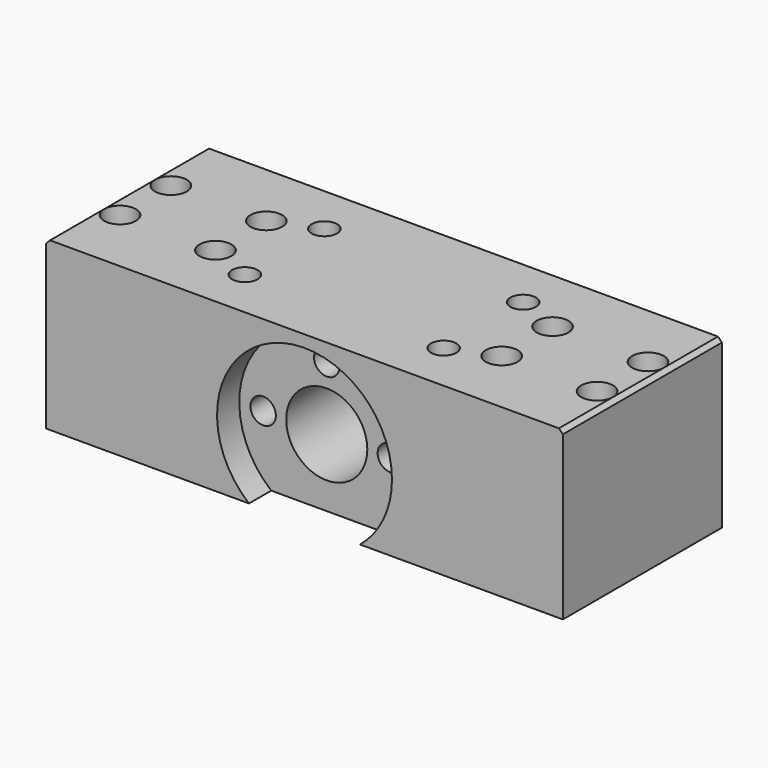
from build123d import *

# Parameters (mm, degrees)
F0_W           = 65
F0_H           = 21
F0_R           = 5.1
F1_DEPTH       = 25
F3_D           = 2.4
F3_CBORE_D     = 4
F3_CBORE_DEPTH = 2.5
F4_SIZE        = 0.49999
F5_R           = 5.1
F6_DEPTH       = 3.5
F8_D           = 3.2
F8_DEPTH       = 8
F8_TIP         = 0.9613769904
F10_D          = 3.2
F10_DEPTH      = 10
F10_TIP        = 0.9613769904
F11_R          = 5.1
F12_DEPTH      = 6


# Not quite as in the source:
# - a fillet or chamfer is up to 0.001 mm smaller than in the source, because OpenCascade refuses the exact size


with BuildPart() as f1:
    # F0 (on Front) → F1 (new body)
    with BuildSketch(Plane.XZ):
        with Locations((0, 2)):
            Rectangle(F0_W, F0_H)
        Circle(F0_R, mode=Mode.SUBTRACT)
    extrude(amount=F1_DEPTH)

    # F3 (through all)
    with Locations(Plane.XY.offset(12.5)):
        with Locations((-30, -8.5), (-30, -16.5), (-18, -8.5), (-18, -16.5), (18, -16.5), (18, -8.5), (30, -8.5), (30, -16.5)):
            CounterBoreHole(F3_D / 2, F3_CBORE_D / 2, F3_CBORE_DEPTH)

    # F4 (size 0.5 in the source; OpenCascade refuses exactly that, so slightly less here)
    f4_edges = [f1.edges().sort_by_distance(p)[0] for p in [
        (-32.5, -12.5, 12.5),
        (32.5, -12.5, 12.5),
    ]]
    chamfer(f4_edges, length=F4_SIZE)

    # F5 (on face) → F6 (cut)
    with BuildSketch(Plane.XZ.offset(25)):
        with BuildLine():
            ThreePointArc((6.9821200219, -8.5), (9.9449313784, -4.7008871375), (11, 0))
            ThreePointArc((11, 0), (-4.7008871375, 9.9449313784), (-6.9821200219, -8.5))
            Line((-6.9821200219, -8.5), (6.9821200219, -8.5))
        make_face()
        Circle(F5_R, mode=Mode.SUBTRACT)
    extrude(amount=-F6_DEPTH, mode=Mode.SUBTRACT)

    # F8
    with Locations(Plane.XY.offset(12.5)):
        with Locations((12.5, -6.25), (12.5, -18.75), (-12.5, -6.25), (-12.5, -18.75)):
            Hole(F8_D / 2, depth=F8_DEPTH)
            with Locations((0, 0, -(F8_DEPTH + F8_TIP / 2))):  # 118° drill point
                Cone(0, F8_D / 2, F8_TIP, mode=Mode.SUBTRACT)

    # F10
    with Locations(Plane.XZ.offset(21.5)):
        with Locations((-8, 0), (0, 8), (8, 0)):
            Hole(F10_D / 2, depth=F10_DEPTH)
            with Locations((0, 0, -(F10_DEPTH + F10_TIP / 2))):  # 118° drill point
                Cone(0, F10_D / 2, F10_TIP, mode=Mode.SUBTRACT)

    # F11 (on face) → F12 (cut)
    with BuildSketch(Plane(origin=(0, 0, 0), x_dir=(-1, 0, 0), z_dir=(0, 1, 0))):
        with BuildLine():
            ThreePointArc((4.2426406871, -8.5), (8.0794519161, -4.9972449146), (9.5, 0))
            ThreePointArc((9.5, 0), (-4.9972449146, 8.0794519161), (-4.2426406871, -8.5))
            Line((-4.2426406871, -8.5), (4.2426406871, -8.5))
        make_face()
        Circle(F11_R, mode=Mode.SUBTRACT)
        Circle(F11_R)
    extrude(amount=-F12_DEPTH, mode=Mode.SUBTRACT)


solid = f1.part
